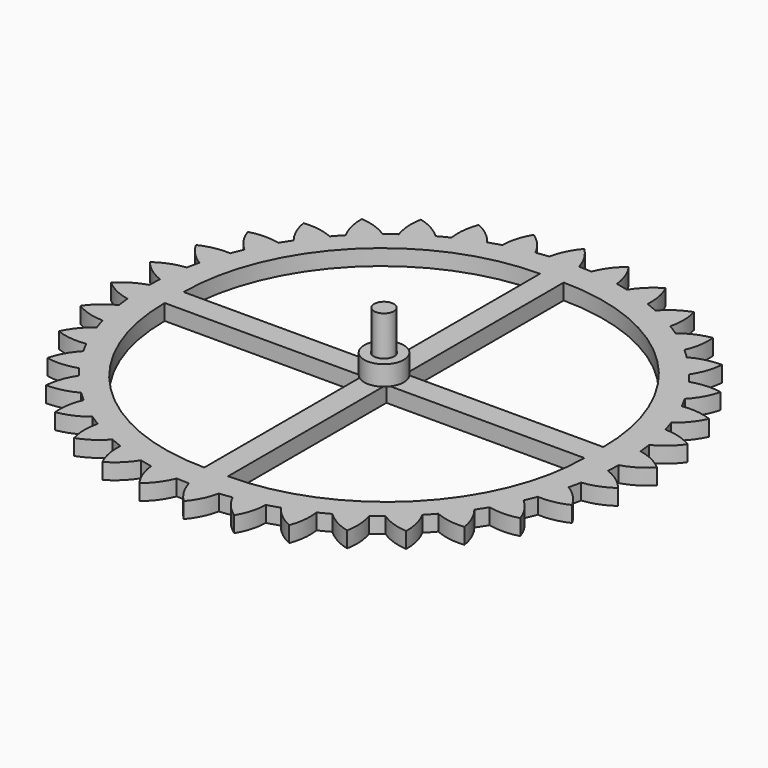
from build123d import *

# Parameters (mm, degrees)
F0_R      = 76.454
F1_DEPTH  = 5.08
F3_DEPTH  = 5.08
F4_COUNT  = 36
F6_DEPTH  = 5.081
F7_R      = 3.175
F8_DEPTH  = 19.05
F9_R      = 6.35
F9_R_2    = 3.302
F10_DEPTH = 6.35


with BuildPart() as f1:
    # F0 (on Top) → F1 (new body)
    with BuildSketch(Plane.XY):
        Circle(F0_R)
    extrude(amount=F1_DEPTH)

    # F2 (on face) → F3 (join, through all)
    with BuildSketch(Plane.XY.offset(5.08)):
        with BuildLine():
            Line((-8.1878878831, 73.2035114732), (2.0336598434, 73.6319212546))
            ThreePointArc((2.0336598434, 73.6319212546), (0.1770309744, 79.6658719085), (-3.5496429493, 84.7617067486))
            Line((-3.5496429493, 84.7617067486), (-3.5554829661, 84.7614619794))
            ThreePointArc((-3.5554829661, 84.7614619794), (-6.8426784504, 79.3716589126), (-8.1878878831, 73.2035114732))
        make_face()
    extrude(amount=-F3_DEPTH)

    # F4: F1 ×36 about axis
    f4_axis = Axis((0, 0, 5.08), (0, 0, 1))


with BuildPart() as f1_1:
    add(f1.part)
    for i in range(1, F4_COUNT):
        add(f1.part.rotate(f4_axis, i * 360 / F4_COUNT))

    # F5 (on face) → F6 (cut, through all)
    with BuildSketch(Plane.XY.offset(5.08)):
        with BuildLine():
            Line((-67.31, 3.81), (-3.81, 3.81))
            Line((-3.81, 3.81), (-3.81, 67.31))
            ThreePointArc((-3.81, 67.31), (-48.7112806053, 48.7112806053), (-67.31, 3.81))
        make_face()
        with BuildLine():
            Line((-3.81, -3.81), (-67.31, -3.81))
            ThreePointArc((-67.31, -3.81), (-48.7112806053, -48.7112806053), (-3.81, -67.31))
            Line((-3.81, -67.31), (-3.81, -3.81))
        make_face()
        with BuildLine():
            Line((3.81, -3.81), (3.81, -67.31))
            ThreePointArc((3.81, -67.31), (48.7112806053, -48.7112806053), (67.31, -3.81))
            Line((67.31, -3.81), (3.81, -3.81))
        make_face()
        with BuildLine():
            Line((3.81, 3.81), (67.31, 3.81))
            ThreePointArc((67.31, 3.81), (48.7112806053, 48.7112806053), (3.81, 67.31))
            Line((3.81, 67.31), (3.81, 3.81))
        make_face()
    extrude(amount=-F6_DEPTH, mode=Mode.SUBTRACT)

    # F7 (on face) → F8 (join)
    with BuildSketch(Plane.XY.offset(5.08)):
        Circle(F7_R)
    extrude(amount=F8_DEPTH)


with BuildPart() as f10:
    # F9 (on face) → F10 (new body)
    with BuildSketch(Plane.XY.offset(5.08)):
        Circle(F9_R)
        Circle(F9_R_2, mode=Mode.SUBTRACT)
    extrude(amount=F10_DEPTH)


solid = Compound([f1_1.part, f10.part])
